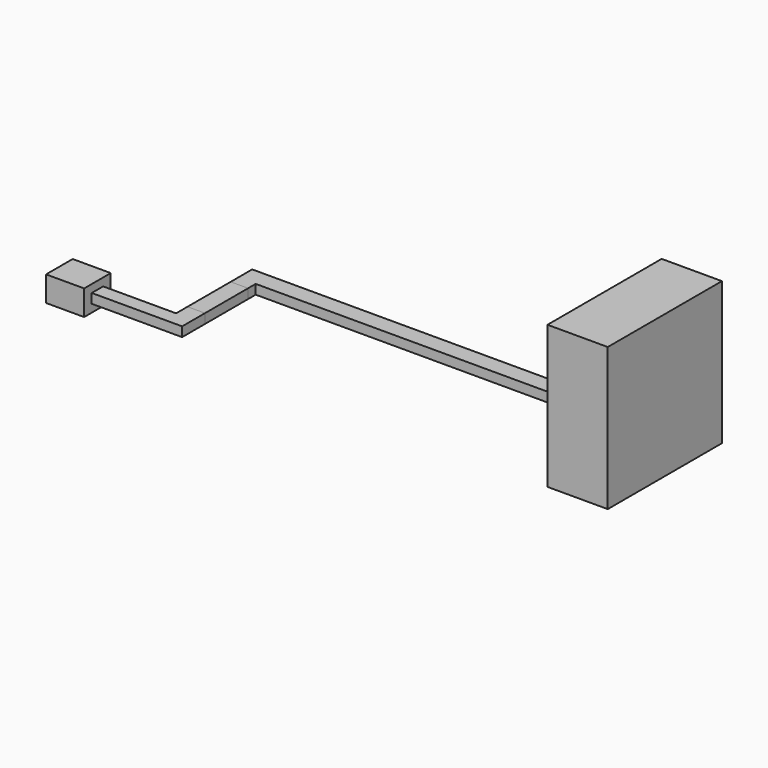
from build123d import *

# Parameters (mm, degrees)
F0_W          = 965.2
F0_H          = 2286
F1_DEPTH      = 2286
F2_W          = 127
F2_H          = 279.4
F3_DEPTH      = 304.8
F4_W          = 279.4
F4_H          = 152.4
F5_DEPTH      = 2286
F6_DEPTH      = 2286
F7_DEPTH      = 1016
F8_W          = 279.4
F8_H          = 152.4
F9_DEPTH      = 152.4
F10_DEPTH     = 863.6
F11_DEPTH     = 457.2
F12_W         = 228.6
F12_H         = 152.4
F13_DEPTH     = 1778
F14_W         = 532.6590749741
F14_H         = 403.9546158791
F14_W_2       = 228.6
F14_H_2       = 152.4
F15_DEPTH     = 609.6
F16_TEXT_SIZE = 501.0474059317
F17_DEPTH     = 5.08


# Not quite as in the source:
# - Text() gives the source's letters only with a copy of the font that has no kerning and outlines rounded to 1/6400 em; it was checked with that copy


with BuildPart() as f1:
    # F0 (on Top) → F1 (new body)
    with BuildSketch(Plane.XY):
        with Locations((482.6, -1143)):
            Rectangle(F0_W, F0_H)
    extrude(amount=F1_DEPTH)

    # F16 (on face) → F17 (join)
    with BuildSketch(Plane(origin=(0, 0, 0), x_dir=(0, -1, 0), z_dir=(-1, 0, 0))):
        with Locations((242.9870516062, 1632.8017711639)):
            Text('MDP-L', F16_TEXT_SIZE, font='Open Sans', text_align=(TextAlign.LEFT, TextAlign.BOTTOM))
    extrude(amount=F17_DEPTH)


with BuildPart() as f3:
    # F2 (on Top) → F3 (new body)
    with BuildSketch(Plane.XY):
        with Locations((-546.6818680763, -589.5562127113)):
            Rectangle(F2_W, F2_H)
    extrude(amount=F3_DEPTH)

    # F4 (on face) → F5 (join)
    with BuildSketch(Plane(origin=(-610.1818680763, 0, 0), x_dir=(0, -1, 0), z_dir=(-1, 0, 0))):
        with Locations((589.5562127113, 228.6)):
            Rectangle(F4_W, F4_H)
    extrude(amount=F5_DEPTH)

    # F6 (add): a face of the model
    f6_faces = [f3.faces().sort_by_distance(p)[0] for p in [
        (-2896.1818680763, -589.5562127113, 228.6),
    ]]
    extrude(f6_faces, amount=F6_DEPTH)

    # F7 (add): a face of the model
    f7_faces = [f3.faces().sort_by_distance(p)[0] for p in [
        (-5182.1818680763, -589.5562127113, 228.6),
    ]]
    extrude(f7_faces, amount=F7_DEPTH)

    # F8 (on face) → F9 (join)
    with BuildSketch(Plane.XZ.offset(729.2562127113)):
        with Locations((-6058.4818680763, 228.6)):
            Rectangle(F8_W, F8_H)
    extrude(amount=F9_DEPTH)


with BuildPart() as f10:
    # F10 (new): a face of the model
    f10_faces = [f3.part.faces().sort_by_distance(p)[0] for p in [
        (-6058.4818680763, -881.6562127113, 228.6),
    ]]
    extrude(f10_faces, amount=F10_DEPTH)


with BuildPart() as f11:
    # F11 (new): a face of the model
    f11_faces = [f10.part.faces().sort_by_distance(p)[0] for p in [
        (-6058.4818680763, -1745.2562127113, 228.6),
    ]]
    extrude(f11_faces, amount=F11_DEPTH)

    # F12 (on face) → F13 (join)
    with BuildSketch(Plane(origin=(-6198.1818680763, 0, 0), x_dir=(0, -1, 0), z_dir=(-1, 0, 0))):
        with Locations((2088.1562127113, 228.6)):
            Rectangle(F12_W, F12_H)
    extrude(amount=F13_DEPTH)

    # F14 (on face) → F15 (join)
    with BuildSketch(Plane(origin=(-7976.1818680763, 0, 0), x_dir=(0, -1, 0), z_dir=(-1, 0, 0))):
        with Locations((2088.1562127113, 228.6)):
            Rectangle(F14_W, F14_H)
        with Locations((2088.1562127113, 228.6)):
            Rectangle(F14_W_2, F14_H_2, mode=Mode.SUBTRACT)
    extrude(amount=-F15_DEPTH)


solid = Compound([f1.part, f3.part, f10.part, f11.part])
